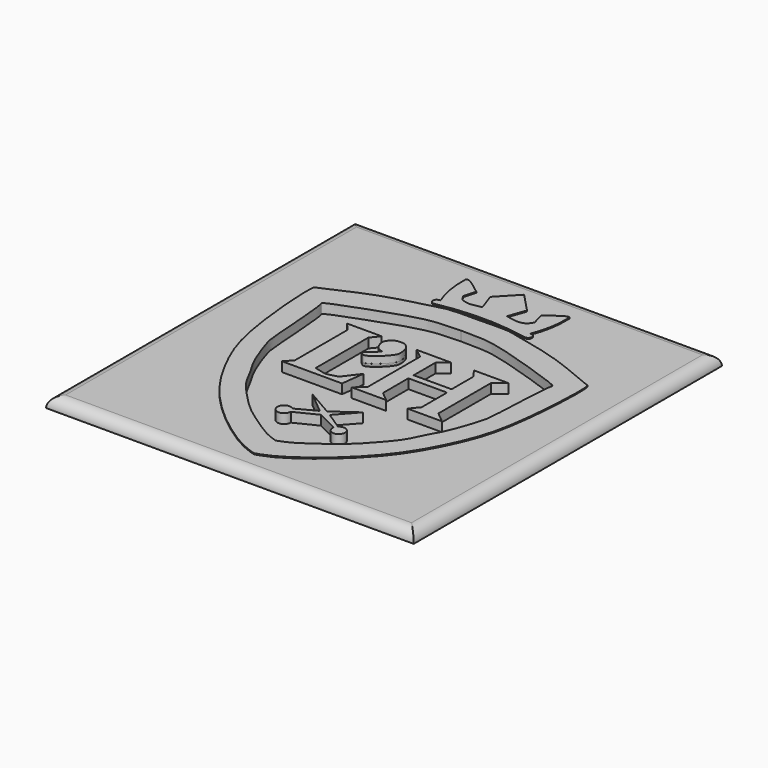
from build123d import *

# Parameters (mm, degrees)
F1_DEPTH    = 5.5
F2_DEPTH    = 5.5
F3_DEPTH    = 2.286
F4_DEPTH    = 5.5
F5_DEPTH    = 5.5
F6_DEPTH    = 1.016
F7_DEPTH    = 5
F8_T1_DEPTH = 197.6471443936
F8_T3_DEPTH = 205.9150099099
F9_DEPTH    = 5.5


# Not quite as in the source:
# - a fillet or chamfer that OpenCascade refuses, or shapes differently, is made with other operations: its cross-section is extruded or revolved along the edge and cut away or added


with BuildPart() as f1:
    # F0 (on Top) → F1 (new body)
    with BuildSketch(Plane.XY):
        with BuildLine():
            ThreePointArc((-23.3652070165, 162.2018367052), (-22.7085829384, 153.0724974029), (-20.1373938471, 144.2881375551))
            ThreePointArc((-20.1373938471, 144.2881375551), (-22.2764581314, 142.6060646772), (-20.1373938471, 140.9239917994))
            ThreePointArc((-20.1373938471, 140.9239917994), (0.8642266621, 142.9842195339), (21.8658471713, 140.9239917994))
            ThreePointArc((21.8658471713, 140.9239917994), (24.0049114555, 142.6060646772), (21.8658471713, 144.2881375551))
            ThreePointArc((21.8658471713, 144.2881375551), (24.4370362625, 153.0724974029), (25.0936603406, 162.2018367052))
            add(Edge.make_bspline(
                [(25.0936603406, 162.2018367052), (25.1603577708, 162.5948878077), (25.2908985179, 163.3641705891), (23.6522805321, 163.9085586719), (19.3248651111, 160.5309974132), (16.0219777608, 157.9530835152)],
                knots=[0, 0, 0, 0, 0.1982919839, 0.3880986669, 1, 1, 1, 1], degree=3))
            Line((16.0219777608, 157.9530835152), (17.6296165446, 152.2115021944))
            Line((17.6296165446, 152.2115021944), (16.0219777608, 149.8000472784))
            add(Edge.make_bspline(
                [(16.0219777608, 149.8000472784), (15.0426324197, 149.3820081262), (12.7224041657, 148.3916054444), (8.8460069058, 149.284205092), (6.605798495, 149.8000472784)],
                knots=[0, 0, 0, 0, 0.422090085, 1, 1, 1, 1], degree=3))
            Line((6.605798495, 149.8000472784), (9.4765840331, 157.9530835152))
            Line((9.4765840331, 157.9530835152), (0.8642266621, 167.0247614384))
            Line((0.8642266621, 167.0247614384), (-7.7481307089, 157.9530835152))
            Line((-7.7481307089, 157.9530835152), (-4.8773451708, 149.8000472784))
            add(Edge.make_bspline(
                [(-14.2935244367, 149.8000472784), (-13.3141790956, 149.3820081262), (-10.9939508415, 148.3916054444), (-7.1175535816, 149.284205092), (-4.8773451708, 149.8000472784)],
                knots=[0, 0, 0, 0, 0.422090085, 1, 1, 1, 1], degree=3))
            Line((-14.2935244367, 149.8000472784), (-15.9011632204, 152.2115021944))
            Line((-15.9011632204, 152.2115021944), (-14.2935244367, 157.9530835152))
            add(Edge.make_bspline(
                [(-23.3652070165, 162.2018367052), (-23.4319044466, 162.5948878077), (-23.5624451938, 163.3641705891), (-21.9238272079, 163.9085586719), (-17.5964117869, 160.5309974132), (-14.2935244367, 157.9530835152)],
                knots=[0, 0, 0, 0, 0.1982919839, 0.3880986669, 1, 1, 1, 1], degree=3))
        make_face()
    extrude(amount=F1_DEPTH)


with BuildPart() as f2:
    # F0 (on Top) → F2 (new body)
    with BuildSketch(Plane.XY):
        with BuildLine():
            add(Edge.make_bspline(
                [(0, 7.9060420394), (-1.5699382556, 8.4554715927), (-5.8163851147, 9.9415958987), (-20.1053538125, 18.9596508578), (-39.5124316854, 36.847272112), (-52.198501167, 58.9000037009), (-60.8963978085, 80.8356161818), (-64.0138277233, 124.0946586031), (-61.3529905011, 123.6764543777), (-41.1983104142, 134.3674625854), (-17.4184192851, 139.295530782), (-13.5792100492, 140.9577877449), (-5.3299707349, 140.9291190051), (0, 140.9105956554)],
                knots=[0, 0, 0, 0, 0.0532913836, 0.1441451775, 0.2610358104, 0.3714146381, 0.4899039426, 0.6299639685, 0.6542878323, 0.7603412932, 0.8726910044, 0.9177435403, 1, 1, 1, 1], degree=3))
            Line((0, 7.9060420394), (2.2081230026, 7.2567099962))
            Line((2.2081230026, 7.2567099962), (4.3975972313, 7.9663873164))
            add(Edge.make_bspline(
                [(4.3975972313, 7.9663873164), (5.9518682846, 8.5586882984), (10.1559377178, 10.1607733712), (24.1920752941, 19.5675147642), (43.1010185153, 37.9809210746), (55.1771955218, 60.3734483624), (63.2699150586, 82.5394672065), (65.1991650272, 125.8677618307), (62.5508050112, 125.3767030528), (42.110358012, 135.5106515614), (18.2041971286, 139.7843560525), (14.3208219986, 141.3406411702), (6.0754754569, 141.0856282928), (0.7480199071, 140.9208602309)],
                knots=[0, 0, 0, 0, 0.0532913836, 0.1441451775, 0.2610358104, 0.3714146381, 0.4899039426, 0.6299639685, 0.6542878323, 0.7603412932, 0.8726910044, 0.9177435403, 1, 1, 1, 1], degree=3))
            Line((0.7480199071, 140.9208602309), (0, 140.9105956554))
        make_face()
        with BuildLine():
            add(Edge.make_bspline(
                [(0.518001535, 130.4224961416), (-2.0605111612, 130.3317692282), (-7.121728381, 130.1535418392), (-14.0439228067, 129.5694574518), (-23.9027878023, 126.6855793328), (-32.2793303721, 123.8381348299), (-53.6286550605, 116.1161142905), (-51.8622709762, 114.638097419), (-49.9349728668, 84.1249321666), (-49.1699078725, 79.0141209832), (-43.5110726439, 63.2901144203), (-39.5516546797, 57.8062888655), (-35.8377994676, 49.5014591408), (-29.3784230203, 42.1693741051), (-22.1121627487, 34.7715121532), (-16.7577802904, 30.5866158786), (-8.5157204507, 25.1443040841), (-3.8671316804, 22.0807094809), (0.0417457552, 20.6694353841), (2.0339240122, 19.9512742662)],
                knots=[0, 0, 0, 0, 0.0528320108, 0.1037621703, 0.1626957122, 0.2268122451, 0.3132735954, 0.3337791975, 0.4371100585, 0.4911829824, 0.5659602431, 0.6178321381, 0.6739218648, 0.7348774457, 0.796013011, 0.8470725035, 0.9066259765, 0.9524520221, 1, 1, 1, 1], degree=3))
            add(Edge.make_bspline(
                [(0.518001535, 130.4224961416), (3.0980328346, 130.4025564673), (8.1622348043, 130.363273414), (15.0978497689, 129.9693504495), (25.0321347184, 127.3570804506), (33.4836556667, 124.7405561756), (55.0368299314, 117.6072578517), (53.3116669818, 116.0813288223), (52.222360305, 85.5267687258), (51.5978214437, 80.3968889408), (46.3725757026, 64.5235274355), (42.5651219778, 58.9331223102), (39.0805454626, 50.5295133354), (32.8247898737, 43.0229470717), (25.7642591647, 35.4284881772), (20.526724238, 31.098246125), (12.4371020804, 25.4318256132), (7.8743271388, 22.2418296445), (4.0056461711, 20.7238293306), (2.0339240122, 19.9512742662)],
                knots=[0, 0, 0, 0, 0.0528320108, 0.1037621703, 0.1626957122, 0.2268122451, 0.3132735954, 0.3337791975, 0.4371100585, 0.4911829824, 0.5659602431, 0.6178321381, 0.6739218648, 0.7348774457, 0.796013011, 0.8470725035, 0.9066259765, 0.9524520221, 1, 1, 1, 1], degree=3))
        make_face(mode=Mode.SUBTRACT)
    extrude(amount=F2_DEPTH)


with BuildPart() as f3:
    # F0 (on Top) → F3 (new body)
    with BuildSketch(Plane.XY):
        with BuildLine():
            add(Edge.make_bspline(
                [(-11.4828553051, 109.4735860825), (-12.3423914664, 109.3926663689), (-13.9444822877, 109.0683559614), (-15.5383042507, 107.2391009361), (-16.515419246, 105.3685775384), (-15.6040815711, 102.5036761457), (-14.5987376798, 100.6794278059), (-12.687536283, 99.6559642335), (-10.4735157328, 99.5545920265), (-17.8345913368, 94.3867091007), (-16.2860809094, 93.7374248694), (-14.5362553228, 91.7394795586), (-5.6187623211, 99.7914670242), (-5.5754695798, 103.0889535756), (-5.8576967475, 106.0530782348), (-7.028940816, 107.7950862968), (-8.7748047147, 109.5459329745), (-10.5944176357, 109.5572266842), (-11.4828553051, 109.4735860825)],
                knots=[0, 0, 0, 0, 0.0594644819, 0.1171235639, 0.1710035897, 0.2350781504, 0.2904415469, 0.3470830218, 0.3818704067, 0.4833963276, 0.5166962695, 0.5680909653, 0.6926556284, 0.7632929243, 0.8259278428, 0.8807333853, 0.9385360522, 1, 1, 1, 1], degree=3))
        make_face()
    extrude(amount=F3_DEPTH)


with BuildPart() as f4:
    # F0 (on Top) → F4 (new body)
    with BuildSketch(Plane.XY):
        Polygon((13.6163216084, 108.353190124), (-2.6059825905, 108.353190124), (1.835839008, 104.8769876361), (1.835839008, 73.9773511887), (-2.6059825905, 70.3080222011), (13.6163216084, 70.3080222011), (9.1745005921, 73.9773511887), (9.1745005921, 88.8478010893), (27.286987296, 88.8478010893), (27.286987296, 73.9773511887), (23.9190047462, 69.9003181064), (40.0741286576, 69.9003181064), (35.1387709149, 73.9773511887), (35.1387709149, 104.8769876361), (40.0741286576, 108.7394356728), (23.9190047462, 108.7394356728), (26.9417855889, 104.8769876361), (26.9417855889, 91.9377654791), (9.1745005921, 91.9377654791), (9.1745005921, 104.8769876361), align=None)
    extrude(amount=F4_DEPTH)


with BuildPart() as f5:
    # F0 (on Top) → F5 (new body)
    with BuildSketch(Plane.XY):
        with BuildLine():
            Line((4.8477946044, 48.2198983104), (13.0085184689, 57.352137367))
            Line((13.0085184689, 57.352137367), (2.3245189805, 49.776211381))
            Line((2.3245189805, 49.776211381), (-10.421577841, 57.1148768067))
            Line((-10.421577841, 57.1148768067), (0, 48.4243556857))
            Line((0, 48.4243556857), (-8.964975516, 43.6743039895))
            ThreePointArc((-8.964975516, 43.6743039895), (-13.8543844398, 39.9591893697), (-7.8571367532, 41.2788167596))
            Line((-7.8571367532, 41.2788167596), (2.3245189805, 46.3000014424))
            Line((2.3245189805, 46.3000014424), (12.1737780049, 41.2788167596))
            ThreePointArc((12.1737780049, 41.2788167596), (17.6663145328, 39.2888758057), (13.0085184689, 42.8148874814))
            Line((13.0085184689, 42.8148874814), (4.8477946044, 48.2198983104))
        make_face()
    extrude(amount=F5_DEPTH)


with BuildPart() as f6:
    # F0 (on Top) → F6 (new body)
    with BuildSketch(Plane.XY):
        with BuildLine():
            add(Edge.make_bspline(
                [(0.518001535, 130.4224961416), (3.0980328346, 130.4025564673), (8.1622348043, 130.363273414), (15.0978497689, 129.9693504495), (25.0321347184, 127.3570804506), (33.4836556667, 124.7405561756), (55.0368299314, 117.6072578517), (53.3116669818, 116.0813288223), (52.222360305, 85.5267687258), (51.5978214437, 80.3968889408), (46.3725757026, 64.5235274355), (42.5651219778, 58.9331223102), (39.0805454626, 50.5295133354), (32.8247898737, 43.0229470717), (25.7642591647, 35.4284881772), (20.526724238, 31.098246125), (12.4371020804, 25.4318256132), (7.8743271388, 22.2418296445), (4.0056461711, 20.7238293306), (2.0339240122, 19.9512742662)],
                knots=[0, 0, 0, 0, 0.0528320108, 0.1037621703, 0.1626957122, 0.2268122451, 0.3132735954, 0.3337791975, 0.4371100585, 0.4911829824, 0.5659602431, 0.6178321381, 0.6739218648, 0.7348774457, 0.796013011, 0.8470725035, 0.9066259765, 0.9524520221, 1, 1, 1, 1], degree=3))
            add(Edge.make_bspline(
                [(0.518001535, 130.4224961416), (-2.0605111612, 130.3317692282), (-7.121728381, 130.1535418392), (-14.0439228067, 129.5694574518), (-23.9027878023, 126.6855793328), (-32.2793303721, 123.8381348299), (-53.6286550605, 116.1161142905), (-51.8622709762, 114.638097419), (-49.9349728668, 84.1249321666), (-49.1699078725, 79.0141209832), (-43.5110726439, 63.2901144203), (-39.5516546797, 57.8062888655), (-35.8377994676, 49.5014591408), (-29.3784230203, 42.1693741051), (-22.1121627487, 34.7715121532), (-16.7577802904, 30.5866158786), (-8.5157204507, 25.1443040841), (-3.8671316804, 22.0807094809), (0.0417457552, 20.6694353841), (2.0339240122, 19.9512742662)],
                knots=[0, 0, 0, 0, 0.0528320108, 0.1037621703, 0.1626957122, 0.2268122451, 0.3132735954, 0.3337791975, 0.4371100585, 0.4911829824, 0.5659602431, 0.6178321381, 0.6739218648, 0.7348774457, 0.796013011, 0.8470725035, 0.9066259765, 0.9524520221, 1, 1, 1, 1], degree=3))
        make_face()
        with BuildLine():
            Line((2.3245189805, 49.776211381), (13.0085184689, 57.352137367))
            Line((13.0085184689, 57.352137367), (4.8477946044, 48.2198983104))
            Line((4.8477946044, 48.2198983104), (13.0085184689, 42.8148874814))
            ThreePointArc((13.0085184689, 42.8148874814), (17.6663145328, 39.2888758057), (12.1737780049, 41.2788167596))
            Line((12.1737780049, 41.2788167596), (2.3245189805, 46.3000014424))
            Line((2.3245189805, 46.3000014424), (-7.8571367532, 41.2788167596))
            ThreePointArc((-7.8571367532, 41.2788167596), (-13.8543844398, 39.9591893697), (-8.964975516, 43.6743039895))
            Line((-8.964975516, 43.6743039895), (0, 48.4243556857))
            Line((0, 48.4243556857), (-10.421577841, 57.1148768067))
            Line((-10.421577841, 57.1148768067), (2.3245189805, 49.776211381))
        make_face(mode=Mode.SUBTRACT)
        with BuildLine():
            Line((-32.1537517011, 104.8769876361), (-35.43683514, 108.7394356728))
            Line((-35.43683514, 108.7394356728), (-19.2145332694, 108.7394356728))
            Line((-19.2145332694, 108.7394356728), (-22.4052499804, 104.8769876361))
            Line((-22.4052499804, 104.8769876361), (-22.4052499804, 73.9773511887))
            add(Edge.make_bspline(
                [(-22.4052499804, 73.9773511887), (-20.71180454, 73.5248203389), (-17.9646481928, 72.7907116592), (-16.128616981, 72.667364307), (-13.268255203, 73.4750909091), (-11.4896260202, 73.9773511887)],
                knots=[0, 0, 0, 0, 0.3780255904, 0.6132440853, 1, 1, 1, 1], degree=3))
            Line((-11.4896260202, 73.9773511887), (-5.8890683576, 81.3160166144))
            Line((-5.8890683576, 81.3160166144), (-7.2409268469, 70.5011487007))
            Line((-7.2409268469, 70.5011487007), (-35.43683514, 70.5011487007))
            Line((-35.43683514, 70.5011487007), (-32.1537517011, 73.9773511887))
            Line((-32.1537517011, 73.9773511887), (-32.1537517011, 104.8769876361))
        make_face(mode=Mode.SUBTRACT)
        with BuildLine():
            add(Edge.make_bspline(
                [(-11.4828553051, 109.4735860825), (-12.3423914664, 109.3926663689), (-13.9444822877, 109.0683559614), (-15.5383042507, 107.2391009361), (-16.515419246, 105.3685775384), (-15.6040815711, 102.5036761457), (-14.5987376798, 100.6794278059), (-12.687536283, 99.6559642335), (-10.4735157328, 99.5545920265), (-17.8345913368, 94.3867091007), (-16.2860809094, 93.7374248694), (-14.5362553228, 91.7394795586), (-5.6187623211, 99.7914670242), (-5.5754695798, 103.0889535756), (-5.8576967475, 106.0530782348), (-7.028940816, 107.7950862968), (-8.7748047147, 109.5459329745), (-10.5944176357, 109.5572266842), (-11.4828553051, 109.4735860825)],
                knots=[0, 0, 0, 0, 0.0594644819, 0.1171235639, 0.1710035897, 0.2350781504, 0.2904415469, 0.3470830218, 0.3818704067, 0.4833963276, 0.5166962695, 0.5680909653, 0.6926556284, 0.7632929243, 0.8259278428, 0.8807333853, 0.9385360522, 1, 1, 1, 1], degree=3))
        make_face(mode=Mode.SUBTRACT)
        Polygon((1.835839008, 104.8769876361), (-2.6059825905, 108.353190124), (13.6163216084, 108.353190124), (9.1745005921, 104.8769876361), (9.1745005921, 91.9377654791), (26.9417855889, 91.9377654791), (26.9417855889, 104.8769876361), (23.9190047462, 108.7394356728), (40.0741286576, 108.7394356728), (35.1387709149, 104.8769876361), (35.1387709149, 73.9773511887), (40.0741286576, 69.9003181064), (23.9190047462, 69.9003181064), (27.286987296, 73.9773511887), (27.286987296, 88.8478010893), (9.1745005921, 88.8478010893), (9.1745005921, 73.9773511887), (13.6163216084, 70.3080222011), (-2.6059825905, 70.3080222011), (1.835839008, 73.9773511887), align=None, mode=Mode.SUBTRACT)
    extrude(amount=F6_DEPTH)


with BuildPart() as f7:
    # F0 (on Top) → F7 (new body)
    with BuildSketch(Plane.XY):
        Polygon((86.0586119816, 176.3824373484), (-86.1885324121, 176.3824373484), (-86.1885324121, -4.1325725615), (86.0586119816, -4.1325725615), (86.0586119816, 118.9667209983), align=None)
        with BuildLine():
            Line((2.2081230026, 7.2567099962), (0, 7.9060420394))
            add(Edge.make_bspline(
                [(0, 7.9060420394), (-1.5699382556, 8.4554715927), (-5.8163851147, 9.9415958987), (-20.1053538125, 18.9596508578), (-39.5124316854, 36.847272112), (-52.198501167, 58.9000037009), (-60.8963978085, 80.8356161818), (-64.0138277233, 124.0946586031), (-61.3529905011, 123.6764543777), (-41.1983104142, 134.3674625854), (-17.4184192851, 139.295530782), (-13.5792100492, 140.9577877449), (-5.3299707349, 140.9291190051), (0, 140.9105956554)],
                knots=[0, 0, 0, 0, 0.0532913836, 0.1441451775, 0.2610358104, 0.3714146381, 0.4899039426, 0.6299639685, 0.6542878323, 0.7603412932, 0.8726910044, 0.9177435403, 1, 1, 1, 1], degree=3))
            Line((0, 140.9105956554), (0.7480199071, 140.9208602309))
            add(Edge.make_bspline(
                [(4.3975972313, 7.9663873164), (5.9518682846, 8.5586882984), (10.1559377178, 10.1607733712), (24.1920752941, 19.5675147642), (43.1010185153, 37.9809210746), (55.1771955218, 60.3734483624), (63.2699150586, 82.5394672065), (65.1991650272, 125.8677618307), (62.5508050112, 125.3767030528), (42.110358012, 135.5106515614), (18.2041971286, 139.7843560525), (14.3208219986, 141.3406411702), (6.0754754569, 141.0856282928), (0.7480199071, 140.9208602309)],
                knots=[0, 0, 0, 0, 0.0532913836, 0.1441451775, 0.2610358104, 0.3714146381, 0.4899039426, 0.6299639685, 0.6542878323, 0.7603412932, 0.8726910044, 0.9177435403, 1, 1, 1, 1], degree=3))
            Line((4.3975972313, 7.9663873164), (2.2081230026, 7.2567099962))
        make_face(mode=Mode.SUBTRACT)
        with BuildLine():
            ThreePointArc((-20.1373938471, 140.9239917994), (-22.2764581314, 142.6060646772), (-20.1373938471, 144.2881375551))
            ThreePointArc((-20.1373938471, 144.2881375551), (-22.7085829384, 153.0724974029), (-23.3652070165, 162.2018367052))
            add(Edge.make_bspline(
                [(-23.3652070165, 162.2018367052), (-23.4319044466, 162.5948878077), (-23.5624451938, 163.3641705891), (-21.9238272079, 163.9085586719), (-17.5964117869, 160.5309974132), (-14.2935244367, 157.9530835152)],
                knots=[0, 0, 0, 0, 0.1982919839, 0.3880986669, 1, 1, 1, 1], degree=3))
            Line((-14.2935244367, 157.9530835152), (-15.9011632204, 152.2115021944))
            Line((-15.9011632204, 152.2115021944), (-14.2935244367, 149.8000472784))
            add(Edge.make_bspline(
                [(-14.2935244367, 149.8000472784), (-13.3141790956, 149.3820081262), (-10.9939508415, 148.3916054444), (-7.1175535816, 149.284205092), (-4.8773451708, 149.8000472784)],
                knots=[0, 0, 0, 0, 0.422090085, 1, 1, 1, 1], degree=3))
            Line((-4.8773451708, 149.8000472784), (-7.7481307089, 157.9530835152))
            Line((-7.7481307089, 157.9530835152), (0.8642266621, 167.0247614384))
            Line((0.8642266621, 167.0247614384), (9.4765840331, 157.9530835152))
            Line((9.4765840331, 157.9530835152), (6.605798495, 149.8000472784))
            add(Edge.make_bspline(
                [(16.0219777608, 149.8000472784), (15.0426324197, 149.3820081262), (12.7224041657, 148.3916054444), (8.8460069058, 149.284205092), (6.605798495, 149.8000472784)],
                knots=[0, 0, 0, 0, 0.422090085, 1, 1, 1, 1], degree=3))
            Line((16.0219777608, 149.8000472784), (17.6296165446, 152.2115021944))
            Line((17.6296165446, 152.2115021944), (16.0219777608, 157.9530835152))
            add(Edge.make_bspline(
                [(25.0936603406, 162.2018367052), (25.1603577708, 162.5948878077), (25.2908985179, 163.3641705891), (23.6522805321, 163.9085586719), (19.3248651111, 160.5309974132), (16.0219777608, 157.9530835152)],
                knots=[0, 0, 0, 0, 0.1982919839, 0.3880986669, 1, 1, 1, 1], degree=3))
            ThreePointArc((25.0936603406, 162.2018367052), (24.4370362625, 153.0724974029), (21.8658471713, 144.2881375551))
            ThreePointArc((21.8658471713, 144.2881375551), (24.0049114555, 142.6060646772), (21.8658471713, 140.9239917994))
            ThreePointArc((21.8658471713, 140.9239917994), (0.8642266621, 142.9842195339), (-20.1373938471, 140.9239917994))
        make_face(mode=Mode.SUBTRACT)
    extrude(amount=F7_DEPTH)

    # F8: fillet of radius 5.08 on 4 edges, made by hand

    # F8_s2 → F8_t1 (cut)
    with BuildSketch(Plane.YZ.offset(-98.8885324121)):
        with BuildLine():
            ThreePointArc((176.3824373484, -0.08), (174.8945397968, 3.5121024484), (171.3024373484, 5))
            Line((171.3024373484, 5), (176.3824373484, 5))
            Line((176.3824373484, 5), (176.3824373484, -0.08))
        make_face()
        with BuildLine():
            ThreePointArc((0.9474274385, 5), (-2.6446750099, 3.5121024484), (-4.1325725615, -0.08))
            Line((-4.1325725615, -0.08), (-4.1325725615, 5))
            Line((-4.1325725615, 5), (0.9474274385, 5))
        make_face()
    extrude(amount=F8_T1_DEPTH, mode=Mode.SUBTRACT)

    # F8_s4 → F8_t3 (cut)
    with BuildSketch(Plane.XZ.offset(-189.0824373484)):
        with BuildLine():
            ThreePointArc((-81.1085324121, 5), (-84.7006348605, 3.5121024484), (-86.1885324121, -0.08))
            Line((-86.1885324121, -0.08), (-86.1885324121, 5))
            Line((-86.1885324121, 5), (-81.1085324121, 5))
        make_face()
        with BuildLine():
            ThreePointArc((80.9786119816, 5), (84.57071443, 3.5121024484), (86.0586119816, -0.08))
            Line((86.0586119816, -0.08), (86.0586119816, 5))
            Line((86.0586119816, 5), (80.9786119816, 5))
        make_face()
    extrude(amount=F8_T3_DEPTH, mode=Mode.SUBTRACT)


with BuildPart() as f9:
    # F0 (on Top) → F9 (new body)
    with BuildSketch(Plane.XY):
        with BuildLine():
            Line((-19.2145332694, 108.7394356728), (-35.43683514, 108.7394356728))
            Line((-35.43683514, 108.7394356728), (-32.1537517011, 104.8769876361))
            Line((-32.1537517011, 104.8769876361), (-32.1537517011, 73.9773511887))
            Line((-32.1537517011, 73.9773511887), (-35.43683514, 70.5011487007))
            Line((-35.43683514, 70.5011487007), (-7.2409268469, 70.5011487007))
            Line((-7.2409268469, 70.5011487007), (-5.8890683576, 81.3160166144))
            Line((-5.8890683576, 81.3160166144), (-11.4896260202, 73.9773511887))
            add(Edge.make_bspline(
                [(-22.4052499804, 73.9773511887), (-20.71180454, 73.5248203389), (-17.9646481928, 72.7907116592), (-16.128616981, 72.667364307), (-13.268255203, 73.4750909091), (-11.4896260202, 73.9773511887)],
                knots=[0, 0, 0, 0, 0.3780255904, 0.6132440853, 1, 1, 1, 1], degree=3))
            Line((-22.4052499804, 73.9773511887), (-22.4052499804, 104.8769876361))
            Line((-22.4052499804, 104.8769876361), (-19.2145332694, 108.7394356728))
        make_face()
    extrude(amount=F9_DEPTH)


with BuildPart() as f9b:
    # F0 (on Top) → F9, piece 2 (new body)
    with BuildSketch(Plane.XY):
        with BuildLine():
            add(Edge.make_bspline(
                [(-11.4828553051, 109.4735860825), (-12.3423914664, 109.3926663689), (-13.9444822877, 109.0683559614), (-15.5383042507, 107.2391009361), (-16.515419246, 105.3685775384), (-15.6040815711, 102.5036761457), (-14.5987376798, 100.6794278059), (-12.687536283, 99.6559642335), (-10.4735157328, 99.5545920265), (-17.8345913368, 94.3867091007), (-16.2860809094, 93.7374248694), (-14.5362553228, 91.7394795586), (-5.6187623211, 99.7914670242), (-5.5754695798, 103.0889535756), (-5.8576967475, 106.0530782348), (-7.028940816, 107.7950862968), (-8.7748047147, 109.5459329745), (-10.5944176357, 109.5572266842), (-11.4828553051, 109.4735860825)],
                knots=[0, 0, 0, 0, 0.0594644819, 0.1171235639, 0.1710035897, 0.2350781504, 0.2904415469, 0.3470830218, 0.3818704067, 0.4833963276, 0.5166962695, 0.5680909653, 0.6926556284, 0.7632929243, 0.8259278428, 0.8807333853, 0.9385360522, 1, 1, 1, 1], degree=3))
        make_face()
    extrude(amount=F9_DEPTH)


solid = Compound([f1.part, f2.part, f3.part, f4.part, f5.part, f6.part, f7.part, f9.part, f9b.part])
